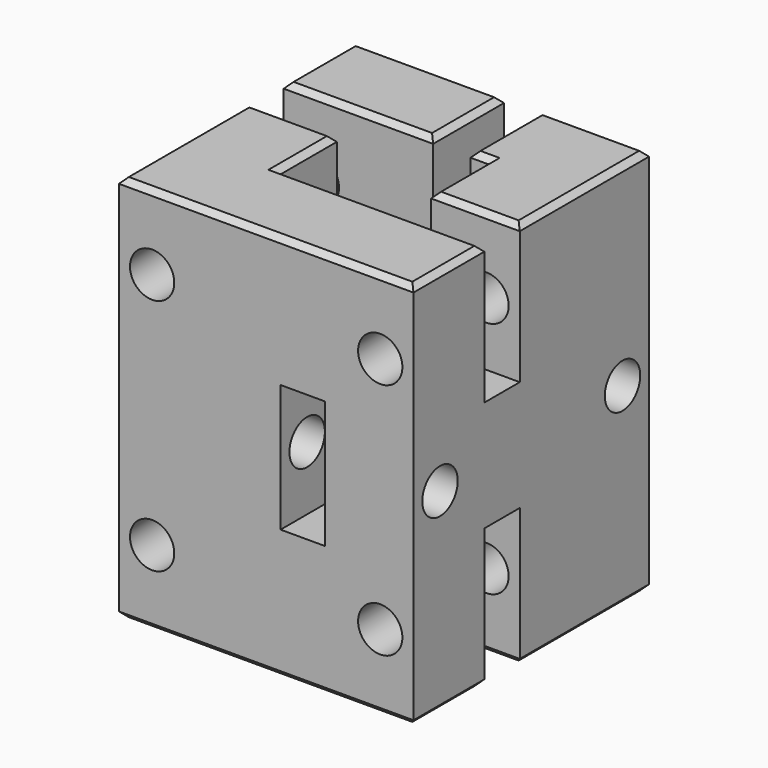
from build123d import *

# Parameters (mm, degrees)
F0_W      = 53.2
F0_H      = 53.2
F0_W_2    = 21.2
F0_H_2    = 21.2
F1_DEPTH  = 70
F2_W      = 8
F2_H      = 7.5
F2_H_2    = 8
F2_H_3    = 2
F4_DEPTH  = 24
F3_W      = 8
F3_H      = 23
F5_DEPTH  = 25
F2_R      = 4
F6_DEPTH  = 90
F7_W      = 8
F7_H      = 7.5
F7_H_2    = 2
F7_H_3    = 8
F8_DEPTH  = 25
F3_R      = 4
F9_DEPTH  = 100
F7_R      = 4
F10_DEPTH = 90
F11_W     = 8
F11_H     = 23
F12_DEPTH = 25
F11_R     = 4
F13_DEPTH = 90
F15_DEPTH = 25
F16_SIZE  = 1


# Not quite as in the source:
# - a feature names something its author has since deleted; it is built from what else it names


with BuildPart() as f1:
    # F0 (on Top) → F1 (new body)
    with BuildSketch(Plane.XY):
        with Locations((-29.3469955068, 26.6660622075)):
            Rectangle(F0_W, F0_H)
        with Locations((-29.3469955068, 26.6660622075)):
            Rectangle(F0_W_2, F0_H_2, mode=Mode.SUBTRACT)
    extrude(amount=F1_DEPTH)

    # F2 (on face) → F4 (cut)
    with BuildSketch(Plane(origin=(-55.9469955068, 0, 0), x_dir=(0, -1, 0), z_dir=(-1, 0, 0))):
        with Locations((-33.2660622075, 48.75)):
            Rectangle(F2_W, F2_H)
        with Locations((-33.2660622075, 56.5)):
            Rectangle(F2_W, F2_H_2)
        with Locations((-33.2660622075, 64.25)):
            Rectangle(F2_W, F2_H)
        with Locations((-33.2660622075, 69)):
            Rectangle(F2_W, F2_H_3)
        with Locations((-33.2660622075, 1)):
            Rectangle(F2_W, F2_H_3)
        with Locations((-33.2660622075, 5.75)):
            Rectangle(F2_W, F2_H)
        with Locations((-33.2660622075, 13.5)):
            Rectangle(F2_W, F2_H_2)
        with Locations((-33.2660622075, 21.25)):
            Rectangle(F2_W, F2_H)
    extrude(amount=-F4_DEPTH, mode=Mode.SUBTRACT)

    # F3 (on face) → F5 (cut)
    with BuildSketch(Plane(origin=(0, 53.2660622075, 0), x_dir=(-1, 0, 0), z_dir=(0, 1, 0))):
        with Locations((35.9469955068, 35)):
            Rectangle(F3_W, F3_H)
    extrude(amount=-F5_DEPTH, mode=Mode.SUBTRACT)

    # F2 (on face) → F6 (cut)
    with BuildSketch(Plane(origin=(-55.9469955068, 0, 0), x_dir=(0, -1, 0), z_dir=(-1, 0, 0))):
        with Locations((-47.2660622075, 35)):
            Circle(F2_R)
    extrude(amount=-F6_DEPTH, mode=Mode.SUBTRACT)

    # F7 (on face) → F8 (cut)
    with BuildSketch(Plane.YZ.offset(-2.7469955068)):
        with Locations((20.0660622075, 48.75)):
            Rectangle(F7_W, F7_H)
        with Locations((20.0660622075, 69)):
            Rectangle(F7_W, F7_H_2)
        with Locations((20.0660622075, 21.25)):
            Rectangle(F7_W, F7_H)
        with Locations((20.0660622075, 1)):
            Rectangle(F7_W, F7_H_2)
        with Locations((20.0660622075, 56.5)):
            Rectangle(F7_W, F7_H_3)
        with Locations((20.0660622075, 64.25)):
            Rectangle(F7_W, F7_H)
        with Locations((20.0660622075, 13.5)):
            Rectangle(F7_W, F7_H_3)
        with Locations((20.0660622075, 5.75)):
            Rectangle(F7_W, F7_H)
    extrude(amount=-F8_DEPTH, mode=Mode.SUBTRACT)

    # F3 (on face) → F9 (cut)
    with BuildSketch(Plane(origin=(0, 53.2660622075, 0), x_dir=(-1, 0, 0), z_dir=(0, 1, 0))):
        with Locations((49.9469955068, 56.5)):
            Circle(F3_R)
        with Locations((49.9469955068, 13.5)):
            Circle(F3_R)
    extrude(amount=-F9_DEPTH, mode=Mode.SUBTRACT)

    # F7 (on face) → F10 (cut)
    with BuildSketch(Plane.YZ.offset(-2.7469955068)):
        with Locations((6.0660622075, 35)):
            Circle(F7_R)
    extrude(amount=-F10_DEPTH, mode=Mode.SUBTRACT)

    # F11 (on face) → F12 (cut)
    with BuildSketch(Plane.XZ.offset(-0.0660622075)):
        with Locations((-22.7469955068, 35)):
            Rectangle(F11_W, F11_H)
    extrude(amount=-F12_DEPTH, mode=Mode.SUBTRACT)

    # F11 (on face) → F13 (cut)
    with BuildSketch(Plane.XZ.offset(-0.0660622075)):
        with Locations((-8.7469955068, 13.5)):
            Circle(F11_R)
        with Locations((-8.7469955068, 56.5)):
            Circle(F11_R)
    extrude(amount=-F13_DEPTH, mode=Mode.SUBTRACT)

    # F14 (on face) → F15 (cut)
    with BuildSketch(Plane(origin=(0, 53.2660622075, 0), x_dir=(-1, 0, 0), z_dir=(0, 1, 0))):
        Polygon((28.9469955068, 0), (22.1969955068, 17.5), (22.1969955068, 0), align=None)
        Polygon((27.4469955068, 35), (22.1969955068, 45.5), (22.1969955068, 24.5), align=None)
        Polygon((28.9469955068, 17.5), (24.8022586647, 17.5), (28.9469955068, 8.75), align=None)
        Polygon((28.9469955068, 52.5), (28.9469955068, 61.25), (24.8022586647, 52.5), align=None)
        Polygon((22.1969955068, 23), (24.8022586647, 17.5), (28.9469955068, 17.5), (28.9469955068, 33.5), align=None)
        Polygon((28.9469955068, 52.5), (24.8022586647, 52.5), (22.1969955068, 47), (28.9469955068, 36.5), align=None)
        Polygon((28.9469955068, 36.5), (22.1969955068, 47), (22.1969955068, 45.5), (27.4469955068, 35), (22.1969955068, 24.5), (22.1969955068, 23), (28.9469955068, 33.5), align=None)
        Polygon((24.8022586647, 17.5), (22.1969955068, 17.5), (28.9469955068, 0), (28.9469955068, 8.75), align=None)
        Polygon((24.8022586647, 52.5), (22.1969955068, 52.5), (22.1969955068, 47), align=None)
        Polygon((22.1969955068, 23), (22.1969955068, 17.5), (24.8022586647, 17.5), align=None)
        Polygon((28.9469955068, 70), (22.1969955068, 70), (22.1969955068, 52.5), align=None)
        Polygon((28.9469955068, 61.25), (28.9469955068, 70), (22.1969955068, 52.5), (24.8022586647, 52.5), align=None)
    extrude(amount=-F15_DEPTH, mode=Mode.SUBTRACT)

    # F16
    f16_edges = [f1.edges().sort_by_distance(p)[0] for p in [
        (-28.946996, 45.266062, 0),
        (-42.446996, 37.266062, 0),
        (-55.946996, 45.266062, 0),
        (-42.446996, 53.266062, 0),
        (-10.746996, 24.066062, 0),
        (-18.746996, 30.666062, 0),
        (-20.471996, 37.266062, 0),
        (-22.196996, 45.266062, 0),
        (-12.471996, 53.266062, 0),
        (-2.746996, 38.666062, 0),
        (-29.346996, 0.066062, 0),
        (-2.746996, 8.066062, 0),
        (-21.346996, 16.066062, 0),
        (-39.946996, 22.666062, 0),
        (-47.946996, 29.266062, 0),
        (-55.946996, 14.666062, 0),
        (-28.946996, 45.266062, 70),
        (-42.446996, 37.266062, 70),
        (-55.946996, 45.266062, 70),
        (-42.446996, 53.266062, 70),
        (-29.346996, 0.066062, 70),
        (-2.746996, 8.066062, 70),
        (-21.346996, 16.066062, 70),
        (-39.946996, 22.666062, 70),
        (-47.946996, 29.266062, 70),
        (-55.946996, 14.666062, 70),
        (-10.746996, 24.066062, 70),
        (-18.746996, 30.666062, 70),
        (-20.471996, 37.266062, 70),
        (-22.196996, 45.266062, 70),
        (-12.471996, 53.266062, 70),
        (-2.746996, 38.666062, 70),
    ]]
    chamfer(f16_edges, length=F16_SIZE)


solid = f1.part
